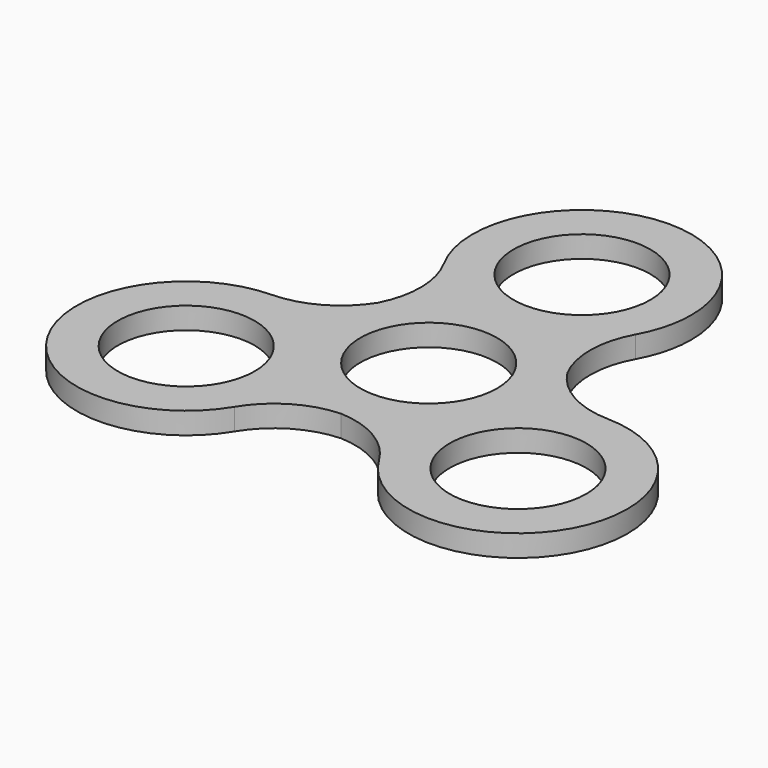
from build123d import *

# Parameters (mm, degrees)
F2_R        = 10
F3_DEPTH    = 1.5875
F4_T1_DEPTH = 3.175


# Not quite as in the source:
# - a fillet or chamfer that OpenCascade refuses, or shapes differently, is made with other operations: its cross-section is extruded or revolved along the edge and cut away or added


with BuildPart() as f3:
    # F2 (on Top) → F3 (new body, symmetric)
    with BuildSketch(Plane.XY):
        with BuildLine():
            ThreePointArc((7.7459666924, 14), (13.7828782748, 19.8739759746), (16, 28))
            ThreePointArc((16, 28), (-8.1260240254, 41.7828782748), (-7.7459666924, 14))
            ThreePointArc((-7.7459666924, 14), (0, 16), (7.7459666924, 14))
        make_face()
        with Locations((0, 28)):
            Circle(F2_R, mode=Mode.SUBTRACT)
        with BuildLine():
            ThreePointArc((7.7459666924, 14), (0, 12), (-7.7459666924, 14))
            ThreePointArc((-7.7459666924, 14), (-13.8564064606, 8), (-15.9973389992, -0.2917960675))
            ThreePointArc((-15.9973389992, -0.2917960675), (-10.3923048454, -6), (-8.2513723068, -13.7082039325))
            ThreePointArc((-8.2513723068, -13.7082039325), (0, -16), (8.2513723068, -13.7082039325))
            ThreePointArc((8.2513723068, -13.7082039325), (10.3923048454, -6), (15.9973389992, -0.2917960675))
            ThreePointArc((15.9973389992, -0.2917960675), (15.999334736, -0.1459041003), (16, 0))
            ThreePointArc((16, 0), (13.7828782748, 8.1260240254), (7.7459666924, 14))
        make_face()
        Circle(F2_R, mode=Mode.SUBTRACT)
        with BuildLine():
            ThreePointArc((-8.2513723068, -13.7082039325), (-13.8564064606, -8), (-15.9973389992, -0.2917960675))
            ThreePointArc((-15.9973389992, -0.2917960675), (-38.1774936811, -21.8733107106), (-8.248711306, -14))
            ThreePointArc((-8.248711306, -14), (-8.24937657, -13.8540958997), (-8.2513723068, -13.7082039325))
        make_face()
        with Locations((-24.248711306, -14)):
            Circle(F2_R, mode=Mode.SUBTRACT)
        with BuildLine():
            ThreePointArc((-8.2513723068, -13.7082039325), (-10.3923048454, -6), (-15.9973389992, -0.2917960675))
            ThreePointArc((-15.9973389992, -0.2917960675), (-13.8564064606, -8), (-8.2513723068, -13.7082039325))
        make_face()
        with BuildLine():
            ThreePointArc((7.7459666924, 14), (0, 16), (-7.7459666924, 14))
            ThreePointArc((-7.7459666924, 14), (0, 12), (7.7459666924, 14))
        make_face()
        with BuildLine():
            ThreePointArc((8.2513723068, -13.7082039325), (13.8564064606, -8), (15.9973389992, -0.2917960675))
            ThreePointArc((15.9973389992, -0.2917960675), (10.3923048454, -6), (8.2513723068, -13.7082039325))
        make_face()
        with BuildLine():
            ThreePointArc((40.248711306, -14), (32.1220220166, -0.0712176249), (15.9973389992, -0.2917960675))
            ThreePointArc((15.9973389992, -0.2917960675), (13.8564064606, -8), (8.2513723068, -13.7082039325))
            ThreePointArc((8.2513723068, -13.7082039325), (24.1028072057, -29.999334736), (40.248711306, -14))
        make_face()
        with Locations((24.248711306, -14)):
            Circle(F2_R, mode=Mode.SUBTRACT)
    extrude(amount=F3_DEPTH, both=True)

    # F4: fillet of radius 13 on 6 edges, made by hand

    # F4_s2 → F4_t1 (join)
    with BuildSketch(Plane.XY.offset(-1.5875)):
        with BuildLine():
            ThreePointArc((14.0120552819, 20.275862069), (12.3968501984, 14), (14.0120552819, 7.724137931))
            ThreePointArc((14.0120552819, 7.724137931), (11.3225214169, 11.3048887108), (7.7459666924, 14))
            ThreePointArc((7.7459666924, 14), (11.3225214169, 16.6951112892), (14.0120552819, 20.275862069))
        make_face()
        with BuildLine():
            ThreePointArc((13.6953273115, 8.2727268678), (18.3227807522, 3.7359871987), (24.5654392763, 1.9968647989))
            ThreePointArc((24.5654392763, 1.9968647989), (20.1196512039, 1.4580355373), (15.9973389992, -0.2917960675))
            ThreePointArc((15.9973389992, -0.2917960675), (15.451581519, 4.1531468265), (13.6953273115, 8.2727268678))
        make_face()
        with BuildLine():
            ThreePointArc((10.5533839944, -22.2727268678), (5.9259305538, -17.7359871987), (-0.3167279703, -15.9968647989))
            ThreePointArc((-0.3167279703, -15.9968647989), (4.1290601021, -15.4580355373), (8.2513723068, -13.7082039325))
            ThreePointArc((8.2513723068, -13.7082039325), (8.797129787, -18.1531468265), (10.5533839944, -22.2727268678))
        make_face()
        with BuildLine():
            ThreePointArc((0.3167279703, -15.9968647989), (-5.9259305538, -17.7359871987), (-10.5533839944, -22.2727268678))
            ThreePointArc((-10.5533839944, -22.2727268678), (-8.797129787, -18.1531468265), (-8.2513723068, -13.7082039325))
            ThreePointArc((-8.2513723068, -13.7082039325), (-4.1290601021, -15.4580355373), (0.3167279703, -15.9968647989))
        make_face()
        with BuildLine():
            ThreePointArc((-24.5654392763, 1.9968647989), (-18.3227807522, 3.7359871987), (-13.6953273115, 8.2727268678))
            ThreePointArc((-13.6953273115, 8.2727268678), (-15.451581519, 4.1531468265), (-15.9973389992, -0.2917960675))
            ThreePointArc((-15.9973389992, -0.2917960675), (-20.1196512039, 1.4580355373), (-24.5654392763, 1.9968647989))
        make_face()
        with BuildLine():
            ThreePointArc((-14.0120552819, 20.275862069), (-12.3968501984, 14), (-14.0120552819, 7.724137931))
            ThreePointArc((-14.0120552819, 7.724137931), (-11.3225214169, 11.3048887108), (-7.7459666924, 14))
            ThreePointArc((-7.7459666924, 14), (-11.3225214169, 16.6951112892), (-14.0120552819, 20.275862069))
        make_face()
    extrude(amount=F4_T1_DEPTH)


solid = f3.part
